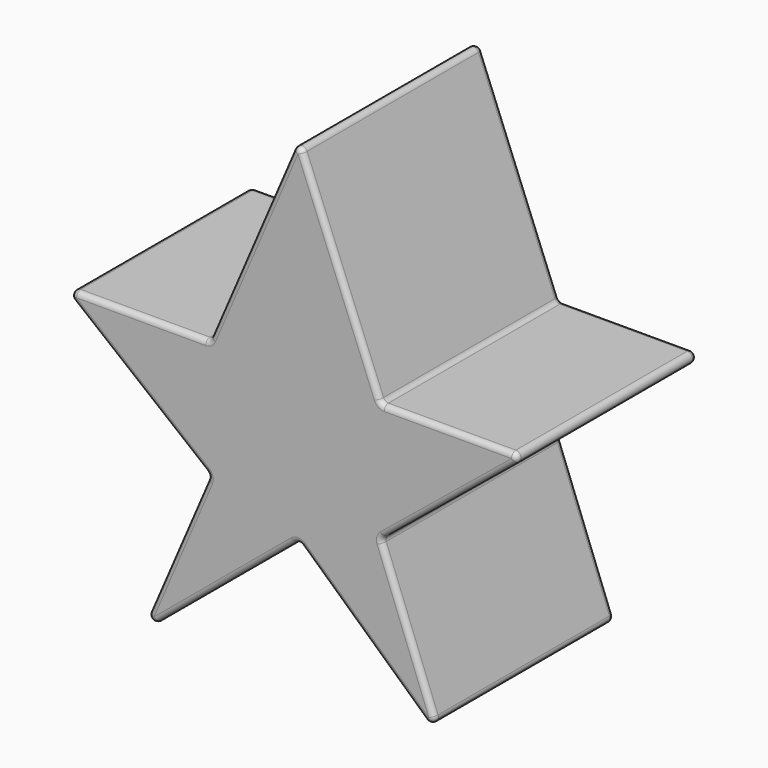
from build123d import *

# Parameters (mm, degrees)
F1_DEPTH = 25.4
F2_R     = 0.6


with BuildPart() as f1:
    # F0 (on Front) → F1 (new body)
    with BuildSketch(Plane.XZ):
        Polygon((9.3241402825, 8.2967067137), (0, 31.6984727979), (-10.0554463643, 8.2967067137), (-26.7336517572, 8.2967067137), (-10.0554463643, -5.155775696), (-17.8360161943, -23.2632836642), (0, -8.402004838), (16.2311457098, -23.2632836642), (9.3241402825, -5.155775696), (25.7989484817, 8.2967067137), align=None)
    extrude(amount=F1_DEPTH)

    # F2
    f2_edges = [f1.edges().sort_by_distance(p)[0] for p in [
        (4.66207, -25.4, 19.99759),
        (-5.027723, -25.4, 19.99759),
        (-18.394549, -25.4, 8.296707),
        (-18.394549, -25.4, 1.570466),
        (-13.945731, -25.4, -14.20953),
        (-8.918008, -25.4, -15.832644),
        (8.115573, -25.4, -15.832644),
        (12.777643, -25.4, -14.20953),
        (17.561544, -25.4, 1.570466),
        (17.561544, -25.4, 8.296707),
        (25.798948, -12.7, 8.296707),
        (9.32414, -12.7, 8.296707),
        (17.561544, 0, 8.296707),
        (0, -12.7, 31.698473),
        (4.66207, 0, 19.99759),
        (-10.055446, -12.7, 8.296707),
        (-5.027723, 0, 19.99759),
        (-10.055446, -12.7, -5.155776),
        (-17.836016, -12.7, -23.263284),
        (-13.945731, 0, -14.20953),
        (-26.733652, -12.7, 8.296707),
        (-18.394549, 0, 1.570466),
        (0, -12.7, -8.402005),
        (16.231146, -12.7, -23.263284),
        (8.115573, 0, -15.832644),
        (-8.918008, 0, -15.832644),
        (9.32414, -12.7, -5.155776),
        (17.561544, 0, 1.570466),
        (12.777643, 0, -14.20953),
        (-18.394549, 0, 8.296707),
    ]]
    fillet(f2_edges, radius=F2_R)


solid = f1.part
